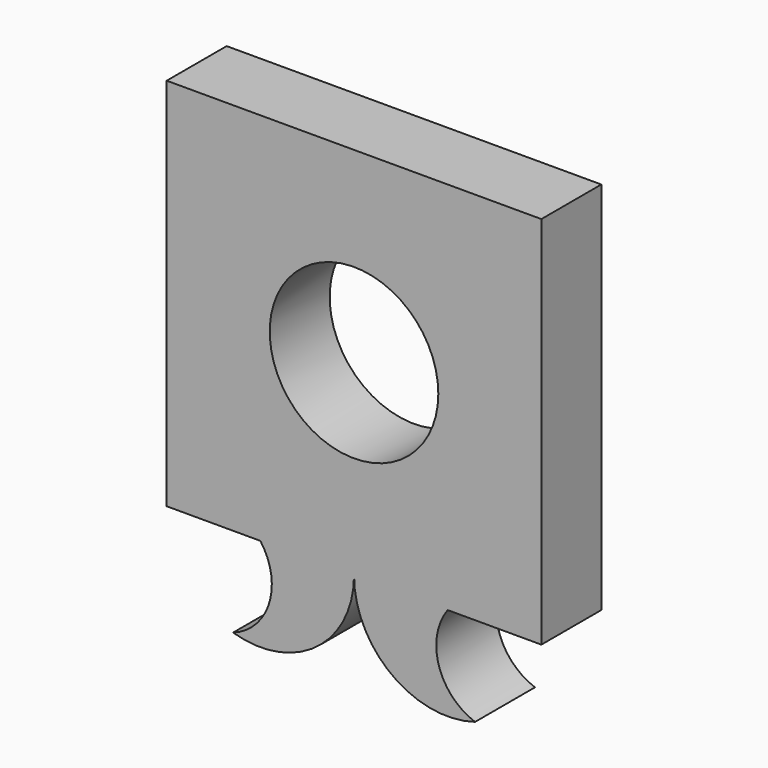
from build123d import *

# Parameters (mm, degrees)
F0_R     = 22.5
F1_DEPTH = 20


# Not quite as in the source:
# - a feature names something its author has since deleted; it is built from what else it names


with BuildPart() as f1:
    # F0 (on Front) → F1 (new body)
    with BuildSketch(Plane.XZ):
        Polygon((37.5, 50), (-40, 50), (-50, 50), (-50, 40), (-50, -40), (-50, -41.9841893017), (-50, -50), (-40, -50), (-25, -50), (0, -50), (25, -50), (40, -50), (50, -50), (50, -41.9841893017), (50, -40), (50, 40), (50, 50), (40, 50), align=None)
        Circle(F0_R, mode=Mode.SUBTRACT)
        with BuildLine():
            ThreePointArc((-25, -50), (-22.6149008919, -63.790810636), (-32.2747059634, -73.9181657563))
            ThreePointArc((-32.2747059634, -73.9181657563), (-10.1149008919, -70.0856621634), (0, -50))
            Line((0, -50), (-25, -50))
        make_face()
        with BuildLine():
            Line((25, -50), (0, -50))
            ThreePointArc((0, -50), (10.1268327857, -70.0944991731), (32.3031117614, -73.909507703))
            ThreePointArc((32.3031117614, -73.909507703), (22.6268327857, -63.7949935854), (25, -50))
        make_face()
    extrude(amount=F1_DEPTH)


solid = f1.part
